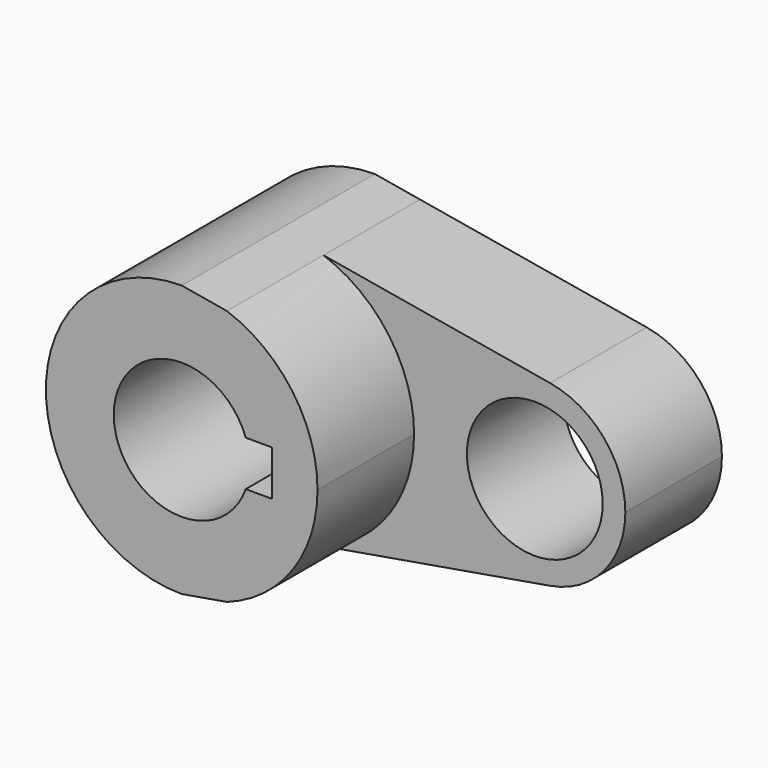
from build123d import *

# Parameters (mm, degrees)
F0_R     = 14.2875
F1_DEPTH = 25.4
F2_DEPTH = 50.8


with BuildPart() as f1:
    # F0 (on Front) → F1 (new body)
    with BuildSketch(Plane.XZ):
        with BuildLine():
            Line((9.5121844836, 26.9452959039), (0, 28.575))
            ThreePointArc((0, 28.575), (-28.575, 0), (0, -28.575))
            Line((0, -28.575), (9.5121844836, -26.9452959039))
            ThreePointArc((9.5121844836, -26.9452959039), (23.3274655355, -16.5033322905), (28.575, 0))
            ThreePointArc((28.575, 0), (23.3274655355, 16.5033322905), (9.5121844836, 26.9452959039))
        make_face()
        with BuildLine():
            ThreePointArc((-13.4703841816, 4.7625), (0, 14.2875), (13.4703841816, 4.7625))
            Line((13.4703841816, 4.7625), (19.05, 4.7625))
            Line((19.05, 4.7625), (19.05, -4.7625))
            Line((19.05, -4.7625), (13.4703841816, -4.7625))
            ThreePointArc((13.4703841816, -4.7625), (0, -14.2875), (-13.4703841816, -4.7625))
            Line((-13.4703841816, -4.7625), (-19.05, -4.7625))
            Line((-19.05, -4.7625), (-19.05, 4.7625))
            Line((-19.05, 4.7625), (-13.4703841816, 4.7625))
        make_face(mode=Mode.SUBTRACT)
        with BuildLine():
            Line((57.1919272622, 18.7764181619), (9.5121844836, 26.9452959039))
            ThreePointArc((9.5121844836, 26.9452959039), (23.3274655355, 16.5033322905), (28.575, 0))
            ThreePointArc((28.575, 0), (23.3274655355, -16.5033322905), (9.5121844836, -26.9452959039))
            Line((9.5121844836, -26.9452959039), (57.1919272622, -18.7764181619))
            ThreePointArc((57.1919272622, -18.7764181619), (34.925, 0), (57.1919272622, 18.7764181619))
        make_face()
        with BuildLine():
            ThreePointArc((73.025, 0), (68.5383952831, 12.2804730295), (57.1919272622, 18.7764181619))
            ThreePointArc((57.1919272622, 18.7764181619), (34.925, 0), (57.1919272622, -18.7764181619))
            ThreePointArc((57.1919272622, -18.7764181619), (68.5383952831, -12.2804730295), (73.025, 0))
        make_face()
        with Locations((53.975, 0)):
            Circle(F0_R, mode=Mode.SUBTRACT)
        with BuildLine():
            ThreePointArc((-13.4703841816, -4.7625), (-14.2875, 0), (-13.4703841816, 4.7625))
            Line((-13.4703841816, 4.7625), (-19.05, 4.7625))
            Line((-19.05, 4.7625), (-19.05, -4.7625))
            Line((-19.05, -4.7625), (-13.4703841816, -4.7625))
        make_face()
    extrude(amount=F1_DEPTH)

    # F0 (on Front) → F2 (join)
    with BuildSketch(Plane.XZ):
        with BuildLine():
            Line((9.5121844836, 26.9452959039), (0, 28.575))
            ThreePointArc((0, 28.575), (-28.575, 0), (0, -28.575))
            Line((0, -28.575), (9.5121844836, -26.9452959039))
            ThreePointArc((9.5121844836, -26.9452959039), (23.3274655355, -16.5033322905), (28.575, 0))
            ThreePointArc((28.575, 0), (23.3274655355, 16.5033322905), (9.5121844836, 26.9452959039))
        make_face()
        with BuildLine():
            ThreePointArc((-13.4703841816, 4.7625), (0, 14.2875), (13.4703841816, 4.7625))
            Line((13.4703841816, 4.7625), (19.05, 4.7625))
            Line((19.05, 4.7625), (19.05, -4.7625))
            Line((19.05, -4.7625), (13.4703841816, -4.7625))
            ThreePointArc((13.4703841816, -4.7625), (0, -14.2875), (-13.4703841816, -4.7625))
            Line((-13.4703841816, -4.7625), (-19.05, -4.7625))
            Line((-19.05, -4.7625), (-19.05, 4.7625))
            Line((-19.05, 4.7625), (-13.4703841816, 4.7625))
        make_face(mode=Mode.SUBTRACT)
        with BuildLine():
            ThreePointArc((-13.4703841816, -4.7625), (-14.2875, 0), (-13.4703841816, 4.7625))
            Line((-13.4703841816, 4.7625), (-19.05, 4.7625))
            Line((-19.05, 4.7625), (-19.05, -4.7625))
            Line((-19.05, -4.7625), (-13.4703841816, -4.7625))
        make_face()
    extrude(amount=F2_DEPTH)


solid = f1.part
